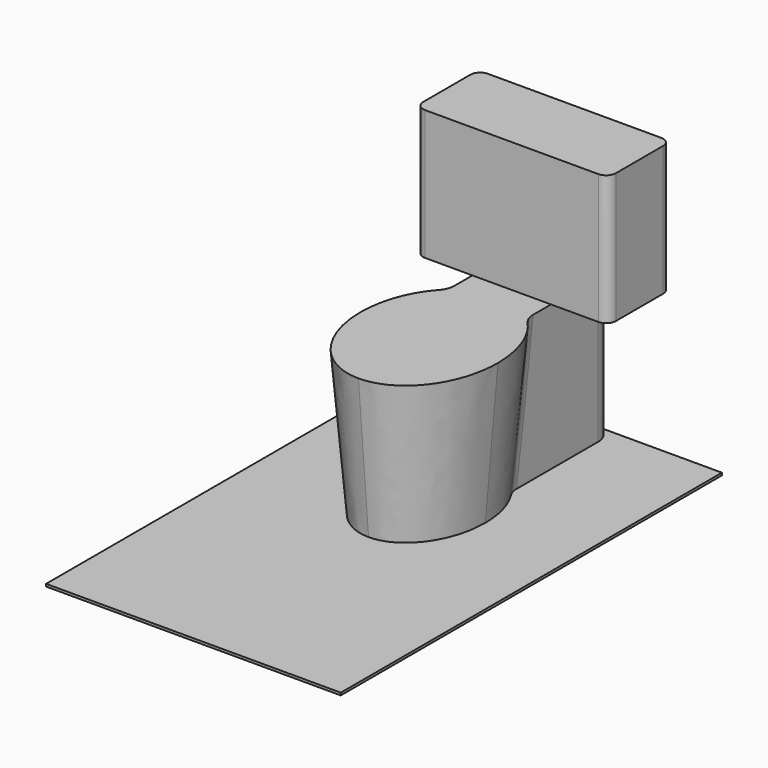
from build123d import *

# Parameters (mm, degrees)
F6_DEPTH  = 381
F6_TAPER  = 5
F7_DEPTH  = 381
F4_W      = 498.475
F4_H      = 203.2
F8_DEPTH  = 336.55
F9_R      = 50.8
F10_R     = 50.8
F11_R     = 25.4
F5_W      = 762
F5_H      = 1231.9
F12_DEPTH = 6.35


with BuildPart() as f6:
    # F2 (on offset) → F6 (new body, through all)
    with BuildSketch(Plane.XY.offset(381)):
        with BuildLine():
            add(Edge.make_bspline(
                [(0, 228.6), (-307.9586335857, 228.6), (-153.9793167929, -114.3), (0, -457.2), (153.9793167929, -114.3), (307.9586335857, 228.6), (0, 228.6)],
                knots=[0, 0, 0, 2.0943951024, 2.0943951024, 4.1887902048, 4.1887902048, 6.2831853072, 6.2831853072, 6.2831853072], degree=2, weights=[1, 0.5, 1, 0.5, 1, 0.5, 1]))
        make_face()
    extrude(amount=-F6_DEPTH, taper=F6_TAPER)

    # F3 (on Top) → F7 (join, through all)
    with BuildSketch(Plane.XY):
        Polygon((-101.6, 469.9), (-101.6, 0), (0, 0), (101.6, 0), (101.6, 469.9), align=None)
    extrude(amount=F7_DEPTH)

    # F4 (on offset) → F8 (join, through all)
    with BuildSketch(Plane.XY.offset(381)):
        with Locations((0, 368.3)):
            Rectangle(F4_W, F4_H)
    extrude(amount=F8_DEPTH)

    # F9
    f9_edges = [f6.edges().sort_by_distance(p)[0] for p in [
        (-101.6, 469.9, 190.5),
        (101.6, 469.9, 190.5),
    ]]
    fillet(f9_edges, radius=F9_R)

    # F10
    f10_edges = [f6.edges().sort_by_distance(p)[0] for p in [
        (101.6, 164.265069, 190.329553),
        (-101.6, 164.265069, 190.329553),
    ]]
    fillet(f10_edges, radius=F10_R)

    # F11
    f11_edges = [f6.edges().sort_by_distance(p)[0] for p in [
        (249.2375, 266.7, 549.275),
        (249.2375, 469.9, 549.275),
        (-249.2375, 266.7, 549.275),
        (-249.2375, 469.9, 549.275),
    ]]
    fillet(f11_edges, radius=F11_R)

    # F5 (on Top) → F12 (join)
    with BuildSketch(Plane.XY):
        with Locations((0, -146.05)):
            Rectangle(F5_W, F5_H)
    extrude(amount=F12_DEPTH)


solid = f6.part
